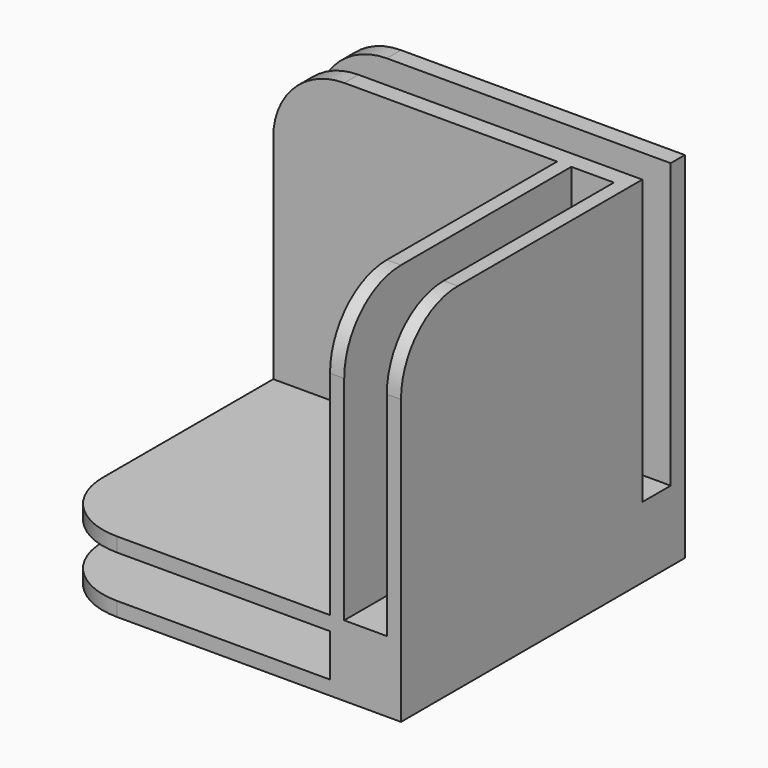
from build123d import *

# Parameters (mm, degrees)
F1_DEPTH = 10
F3_DEPTH = 10
F5_DEPTH = 10
F6_W     = 20
F6_H     = 6
F6_W_2   = 6
F6_H_2   = 30
F6_H_3   = 20
F7_DEPTH = 40
F8_W     = 5
F8_H     = 5
F8_W_2   = 15
F8_W_3   = 40
F9_DEPTH = 40


# Not quite as in the source:
# - a feature names something its author has since deleted; it is built from what else it names


with BuildPart() as f1:
    # F0 (on Top) → F1 (new body)
    with BuildSketch(Plane.XY):
        with BuildLine():
            Line((0, -50), (0, 0))
            Line((0, 0), (-50, 0))
            Line((-50, 0), (-50, -40))
            ThreePointArc((-50, -40), (-47.0710678119, -47.0710678119), (-40, -50))
            Line((-40, -50), (0, -50))
        make_face()
    extrude(amount=F1_DEPTH)

    # F2 (on Right) → F3 (join)
    with BuildSketch(Plane.YZ):
        with BuildLine():
            Line((-50, 10), (0, 10))
            Line((0, 10), (0, 50))
            Line((0, 50), (-40, 50))
            ThreePointArc((-40, 50), (-47.0710678119, 47.0710678119), (-50, 40))
            Line((-50, 40), (-50, 10))
        make_face()
    extrude(amount=-F3_DEPTH)

    # F4 (on Front) → F5 (join)
    with BuildSketch(Plane.XZ):
        with BuildLine():
            Line((-50, 10), (-10, 10))
            Line((-10, 10), (-10, 50))
            Line((-10, 50), (-40, 50))
            ThreePointArc((-40, 50), (-47.0710678119, 47.0710678119), (-50, 40))
            Line((-50, 40), (-50, 10))
        make_face()
    extrude(amount=F5_DEPTH)

    # F6 (on face) → F7 (cut)
    with BuildSketch(Plane.XZ.offset(50)):
        Polygon((-15, 2), (-10, 2), (-10, 8), (-40, 8), (-40, 2), align=None)
        with Locations((-50, 5)):
            Rectangle(F6_W, F6_H)
        with Locations((-5, 25)):
            Rectangle(F6_W_2, F6_H_2)
        with Locations((-5, 50)):
            Rectangle(F6_W_2, F6_H_3)
    extrude(amount=-F7_DEPTH, mode=Mode.SUBTRACT)

    # F8 (on face) → F9 (cut)
    with BuildSketch(Plane.XY.offset(50)):
        with Locations((2.5, -5)):
            Rectangle(F8_W, F8_H)
        with Locations((-47.5, -5)):
            Rectangle(F8_W_2, F8_H)
        with Locations((-20, -5)):
            Rectangle(F8_W_3, F8_H)
    extrude(amount=-F9_DEPTH, mode=Mode.SUBTRACT)


solid = f1.part
